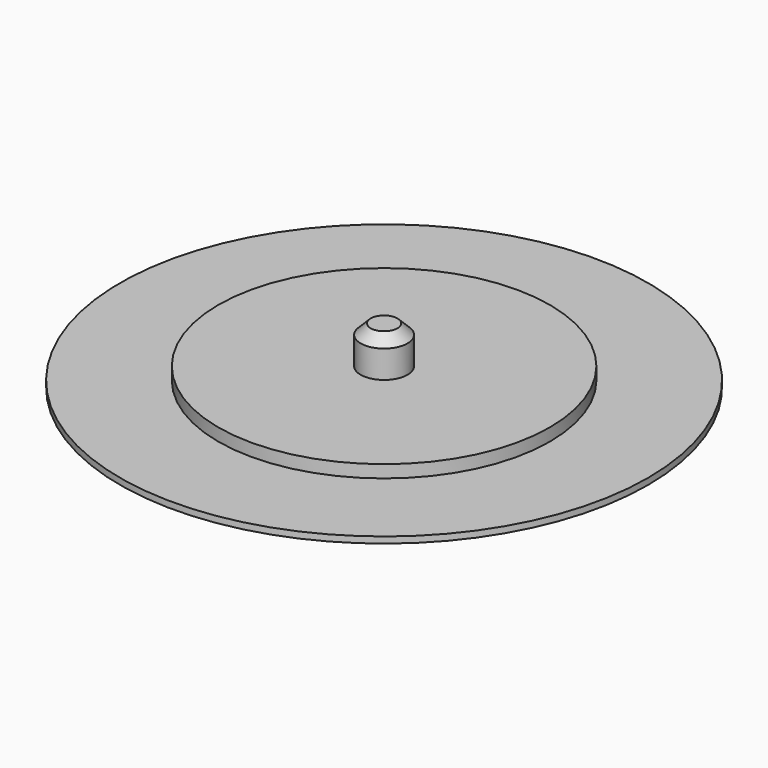
from build123d import *

# Parameters (mm, degrees)
F0_R     = 56.4975790588
F0_R_2   = 10.6711715236
F1_DEPTH = 3.175
F3_R     = 11.8449199959
F4_DEPTH = 25.4
F2_R     = 83.8412354112
F2_R_2   = 56.4975790588
F5_DEPTH = 6.35
F6_SIZE  = 5.08
F7_R     = 133.4753759341
F8_DEPTH = 3.175


with BuildPart() as f1:
    # F0 (on Top) → F1 (new body)
    with BuildSketch(Plane.XY):
        Circle(F0_R)
        Circle(F0_R_2, mode=Mode.SUBTRACT)
        Circle(F0_R_2)
    extrude(amount=F1_DEPTH)

    # F3 (on face) → F4 (join)
    with BuildSketch(Plane.XY.offset(3.175)):
        Circle(F3_R)
    extrude(amount=F4_DEPTH)

    # F2 (on face) → F5 (join)
    with BuildSketch(Plane.XY.offset(3.175)):
        Circle(F2_R)
        Circle(F2_R_2, mode=Mode.SUBTRACT)
        Circle(F2_R_2)
    extrude(amount=F5_DEPTH)

    # F6
    f6_edges = [f1.edges().sort_by_distance(p)[0] for p in [
        (-11.84492, 0, 28.575),
    ]]
    chamfer(f6_edges, length=F6_SIZE)

    # F7 (on Top) → F8 (join)
    with BuildSketch(Plane.XY):
        Circle(F7_R)
    extrude(amount=F8_DEPTH)


solid = f1.part
